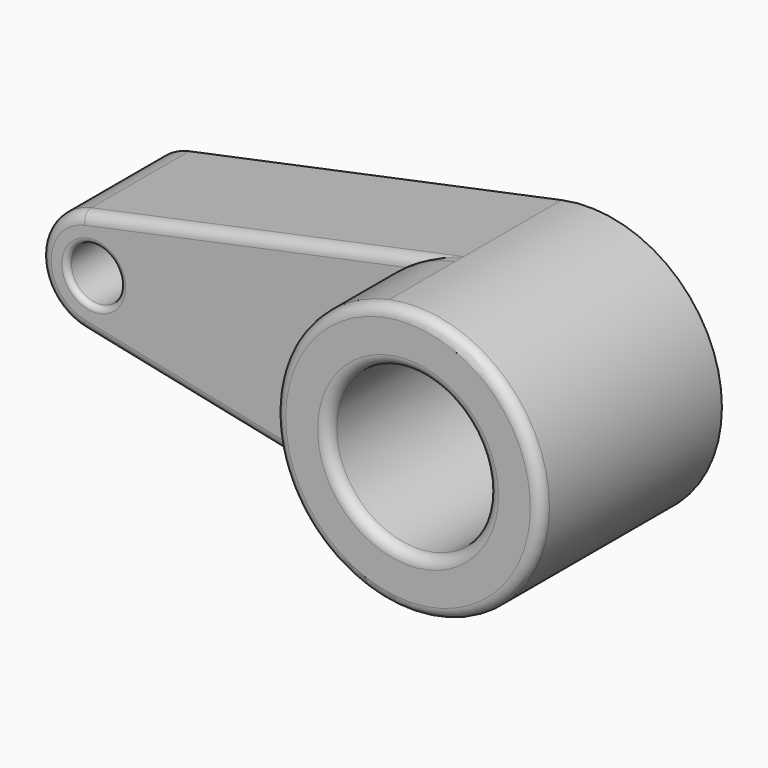
from build123d import *

# Parameters (mm, degrees)
F0_R         = 15
F0_R_2       = 5
F1_DEPTH     = 12.5
F2_DEPTH     = 30
F3_T4_DEPTH  = 86.5228675813
F3_S5_R      = 25
F3_T6_DEPTH  = 45
F3_T8_ANGLE  = 156.3108298238
F3_T12_DEPTH = 86.5228675813
F3_S13_R     = 25
F3_T14_DEPTH = 45
F4_R         = 1


# Not quite as in the source:
# - a fillet or chamfer that OpenCascade refuses, or shapes differently, is made with other operations: its cross-section is extruded or revolved along the edge and cut away or added


with BuildPart() as f1:
    # F0 (on Front) → F1 (new body, symmetric)
    with BuildSketch(Plane.XZ):
        with BuildLine():
            ThreePointArc((-60.0797491716, 17.2713649638), (-51.7234339832, 15.247202645), (-48.0271721521, 7.4842853392))
            ThreePointArc((-48.0271721521, 7.4842853392), (-51.7234339832, -0.2786319667), (-60.0797491716, -2.3027942855))
            Line((-60.0797491716, -2.3027942855), (9.9202508284, -16.9834137224))
            ThreePointArc((9.9202508284, -16.9834137224), (-9.9483066228, 7.4842853392), (9.9202508284, 31.9519844007))
            Line((9.9202508284, 31.9519844007), (-60.0797491716, 17.2713649638))
        make_face()
        with BuildLine():
            ThreePointArc((40.0516933772, 7.4842853392), (30.8110387995, 26.8915786038), (9.9202508284, 31.9519844007))
            ThreePointArc((9.9202508284, 31.9519844007), (-9.9483066228, 7.4842853392), (9.9202508284, -16.9834137224))
            ThreePointArc((9.9202508284, -16.9834137224), (30.8110387995, -11.9230079255), (40.0516933772, 7.4842853392))
        make_face()
        with Locations((15.0516933772, 7.4842853392)):
            Circle(F0_R, mode=Mode.SUBTRACT)
        with BuildLine():
            ThreePointArc((-60.0797491716, -2.3027942855), (-51.7234339832, -0.2786319667), (-48.0271721521, 7.4842853392))
            ThreePointArc((-48.0271721521, 7.4842853392), (-51.7234339832, 15.247202645), (-60.0797491716, 17.2713649638))
            ThreePointArc((-60.0797491716, 17.2713649638), (-68.0271721521, 7.4842853392), (-60.0797491716, -2.3027942855))
        make_face()
        with Locations((-58.0271721521, 7.4842853392)):
            Circle(F0_R_2, mode=Mode.SUBTRACT)
    extrude(amount=F1_DEPTH, both=True)

    # F0 (on Front) → F2 (join)
    with BuildSketch(Plane.XZ):
        with BuildLine():
            ThreePointArc((40.0516933772, 7.4842853392), (30.8110387995, 26.8915786038), (9.9202508284, 31.9519844007))
            ThreePointArc((9.9202508284, 31.9519844007), (-9.9483066228, 7.4842853392), (9.9202508284, -16.9834137224))
            ThreePointArc((9.9202508284, -16.9834137224), (30.8110387995, -11.9230079255), (40.0516933772, 7.4842853392))
        make_face()
        with Locations((15.0516933772, 7.4842853392)):
            Circle(F0_R, mode=Mode.SUBTRACT)
    extrude(amount=F2_DEPTH)

    # F3: fillet of radius 2 on 5 edges, made by hand


with BuildPart() as f3_tool2:
    # F3_s3 → F3_t4 (new body)
    with BuildSketch(Plane(origin=(-57.0859435933, 0, 11.9722430442), x_dir=(0, 1, 0), z_dir=(0.9787079625, 0, -0.205257702))):
        with BuildLine():
            ThreePointArc((-12.5, -12.5855943521), (-11.9142135624, -13.9998079144), (-10.5, -14.5855943521))
            Line((-10.5, -14.5855943521), (-12.5, -14.5855943521))
            Line((-12.5, -14.5855943521), (-12.5, -12.5855943521))
        make_face()
    extrude(amount=F3_T4_DEPTH)

    # F3_s5 → F3_t6 (cut, symmetric)
    with BuildSketch(Plane.XZ.offset(11.5)):
        with Locations((15.0516933772, 7.4842853392)):
            Circle(F3_S5_R)
    extrude(amount=F3_T6_DEPTH, both=True, mode=Mode.SUBTRACT)


with BuildPart() as f1_1:
    add(f1.part)

    # F3_t1: cut F3_tool2
    add(f3_tool2.part, mode=Mode.SUBTRACT)

    # F3_s7 → F3_t8 (revolve, cut)
    with BuildSketch(Plane(origin=(-54.0789471374, 0, -11.3416063211), x_dir=(0, 1, 0), z_dir=(0.9787079625, 0, 0.205257702))):
        with BuildLine():
            ThreePointArc((-10.5, 29.2354536617), (-11.9142135624, 28.649667224), (-12.5, 27.2354536617))
            Line((-12.5, 27.2354536617), (-12.5, 29.2354536617))
            Line((-12.5, 29.2354536617), (-10.5, 29.2354536617))
        make_face()
    revolve(axis=Axis((-58.0271721521, -12.5, 7.4842853392), (0, -1, 0)), revolution_arc=F3_T8_ANGLE, mode=Mode.SUBTRACT)


with BuildPart() as f3_tool10:
    # F3_s11 → F3_t12 (new body)
    with BuildSketch(Plane(origin=(30.6016722995, 0, 6.4178786452), x_dir=(0, 1, 0), z_dir=(-0.9787079625, 0, -0.205257702))):
        with BuildLine():
            ThreePointArc((-10.5, -29.2354536617), (-11.9142135624, -28.649667224), (-12.5, -27.2354536617))
            Line((-12.5, -27.2354536617), (-12.5, -29.2354536617))
            Line((-12.5, -29.2354536617), (-10.5, -29.2354536617))
        make_face()
    extrude(amount=F3_T12_DEPTH)

    # F3_s13 → F3_t14 (cut, symmetric)
    with BuildSketch(Plane.XZ.offset(11.5)):
        with Locations((15.0516933772, 7.4842853392)):
            Circle(F3_S13_R)
    extrude(amount=F3_T14_DEPTH, both=True, mode=Mode.SUBTRACT)


with BuildPart() as f1_2:
    add(f1_1.part)

    # F3_t9: cut F3_tool10
    add(f3_tool10.part, mode=Mode.SUBTRACT)

    # F3_s15 → F3_t16 (revolve, cut)
    with BuildSketch(Plane(origin=(15.9210528626, 0, 3.3390131159), x_dir=(0, 1, 0), z_dir=(-0.9787079625, 0, -0.205257702))):
        with BuildLine():
            ThreePointArc((-28, -29.2354536617), (-29.4142135624, -28.649667224), (-30, -27.2354536617))
            Line((-30, -27.2354536617), (-30, -29.2354536617))
            Line((-30, -29.2354536617), (-28, -29.2354536617))
        make_face()
    revolve(axis=Axis((15.0516933772, -30, 7.4842853392), (0, 1, 0)), mode=Mode.SUBTRACT)

    # F3_s17 → F3_t18 (revolve, cut)
    with BuildSketch(Plane.XY.offset(7.4842853392)):
        with BuildLine():
            ThreePointArc((32.0516933772, -30), (30.6374798149, -29.4142135624), (30.0516933772, -28))
            Line((30.0516933772, -28), (30.0516933772, -30))
            Line((30.0516933772, -30), (32.0516933772, -30))
        make_face()
    revolve(axis=Axis((15.0516933772, -30, 7.4842853392), (0, -1, 0)), mode=Mode.SUBTRACT)

    # F4
    f4_edges = [f1_2.edges().sort_by_distance(p)[0] for p in [
        (-63.027172, -12.5, 7.484285),
    ]]
    fillet(f4_edges, radius=F4_R)


solid = f1_2.part
